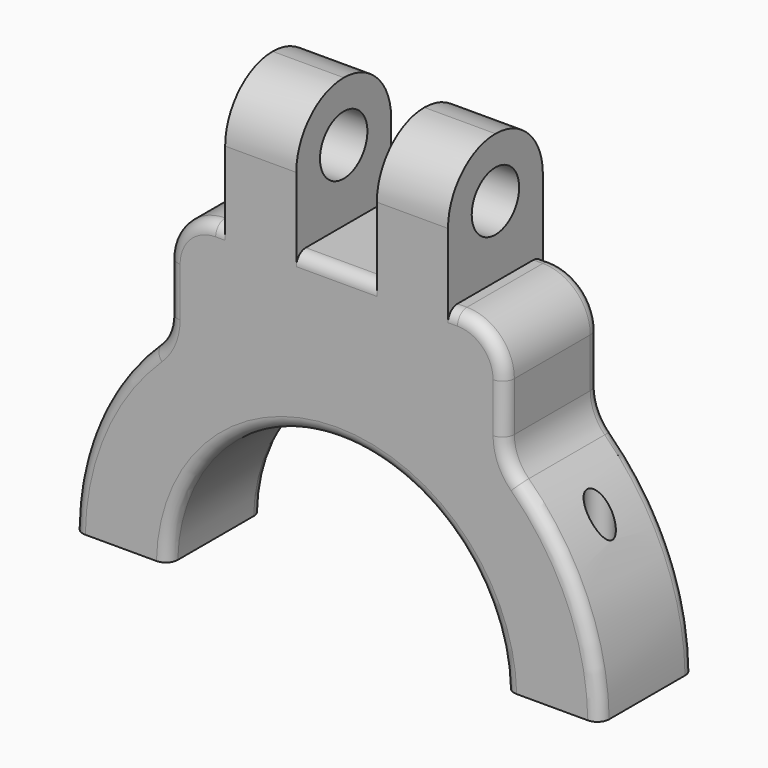
from build123d import *

# Parameters (mm, degrees)
F1_DEPTH  = 12.7
F5_W      = 7.62
F5_H      = 12.7
F6_DEPTH  = 13.97
F8_DEPTH  = 23.876
F9_R      = 6.34999
F10_R     = 5.08
F12_DEPTH = 18.5489899089
F14_DEPTH = 18.5489899089
F15_R     = 1.27


# Not quite as in the source:
# - a fillet or chamfer is up to 0.001 mm smaller than in the source, because OpenCascade refuses the exact size


with BuildPart() as f1:
    # F0 (on Front) → F1 (new body)
    with BuildSketch(Plane.XZ):
        with BuildLine():
            ThreePointArc((56.3854255581, 0.381), (28.194, 28.194), (0.0025744419, 0.381))
            Line((0.0025744419, 0.381), (10.1640250971, 0.381))
            ThreePointArc((10.1640250971, 0.381), (28.194, 18.034), (46.2239749029, 0.381))
            Line((46.2239749029, 0.381), (56.3854255581, 0.381))
        make_face()
    extrude(amount=F1_DEPTH)

    # F3 (on offset) → F4 (join, up to the next surface of F1)
    with BuildSketch(Plane.XY.offset(34.29)):
        Polygon((28.194, 0), (10.16, 0), (10.16, -12.7), (46.228, -12.7), (46.228, 0), align=None)
    extrude(until=Until.NEXT, dir=(0, 0, -1))

    # F5 (on face) → F6 (join)
    with BuildSketch(Plane.XY.offset(34.29)):
        with Locations((20.066, -6.35)):
            Rectangle(F5_W, F5_H)
        with Locations((36.322, -6.35)):
            Rectangle(F5_W, F5_H)
    extrude(amount=F6_DEPTH)

    # F7 (on face) → F8 (cut, through all)
    with BuildSketch(Plane(origin=(16.256, 0, 0), x_dir=(0, -1, 0), z_dir=(-1, 0, 0))):
        with BuildLine():
            ThreePointArc((9.525, 41.91), (8.5950640303, 44.1550640303), (6.35, 45.085))
            ThreePointArc((6.35, 45.085), (4.1049359697, 39.6649359697), (9.525, 41.91))
        make_face()
    extrude(amount=-F8_DEPTH, mode=Mode.SUBTRACT)

    # F9 (radius 6.35 in the source; OpenCascade refuses exactly that, so slightly less here)
    f9_edges = [f1.edges().sort_by_distance(p)[0] for p in [
        (20.066, -12.7, 48.26),
        (20.066, 0, 48.26),
        (36.322, -12.7, 48.26),
        (36.322, 0, 48.26),
    ]]
    fillet(f9_edges, radius=F9_R)

    # F10
    f10_edges = [f1.edges().sort_by_distance(p)[0] for p in [
        (10.16, -6.35, 34.29),
        (10.16, -6.35, 21.672021),
        (46.228, -6.35, 34.29),
        (46.228, -6.35, 21.672021),
    ]]
    fillet(f10_edges, radius=F10_R)

    # F11 (on face) → F12 (cut, up to face)
    with BuildSketch(Plane(origin=(0, 0, 0.381), x_dir=(1, 0, 0), z_dir=(0, 0, -1))):
        with BuildLine():
            ThreePointArc((52.6572502305, 6.35), (52.2610975074, 7.3063972769), (51.3047002305, 7.70255))
            ThreePointArc((51.3047002305, 7.70255), (50.3483029536, 5.3936027231), (52.6572502305, 6.35))
        make_face()
    extrude(amount=-F12_DEPTH, mode=Mode.SUBTRACT)

    # F13 (on face) → F14 (cut, up to face)
    with BuildSketch(Plane(origin=(0, 0, 0.381), x_dir=(1, 0, 0), z_dir=(0, 0, -1))):
        with BuildLine():
            ThreePointArc((6.4358497695, 6.35), (6.0396970464, 7.3063972769), (5.0832997695, 7.70255))
            ThreePointArc((5.0832997695, 7.70255), (4.1269024926, 5.3936027231), (6.4358497695, 6.35))
        make_face()
    extrude(amount=-F14_DEPTH, mode=Mode.SUBTRACT)

    # F15
    f15_edges = [f1.edges().sort_by_distance(p)[0] for p in [
        (28.194, 0, 18.034),
        (2.316329, 0, 11.191416),
        (2.316329, -12.7, 11.191416),
        (28.194, -12.7, 18.034),
        (54.071671, -12.7, 11.191416),
        (54.071671, 0, 11.191416),
        (28.194, 0, 34.29),
        (28.194, -12.7, 34.29),
    ]]
    fillet(f15_edges, radius=F15_R)


solid = f1.part
